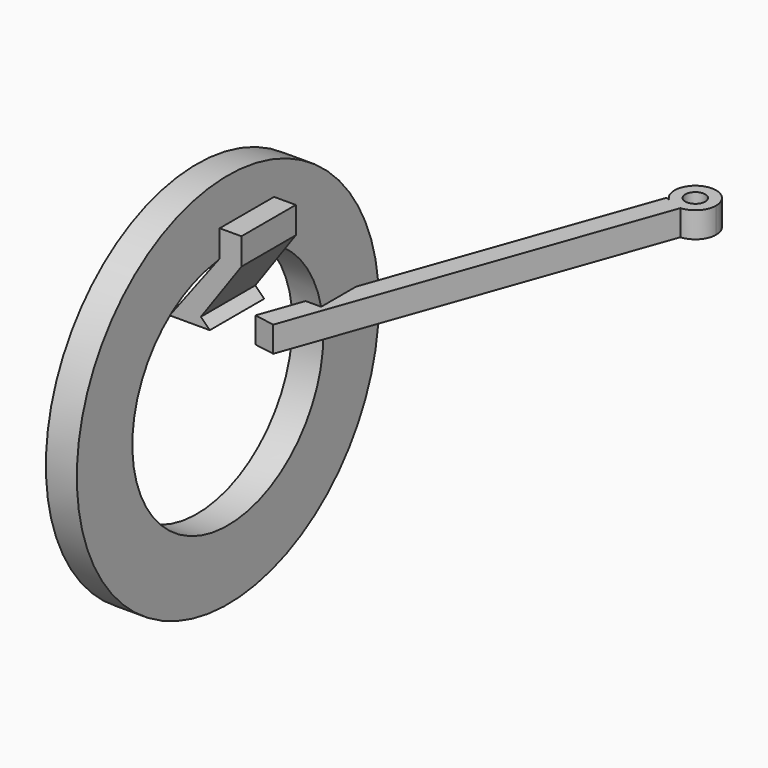
from build123d import *

# Parameters (mm, degrees)
F1_R     = 3.3434072236
F2_DEPTH = 8.636
F0_R     = 63.5
F0_R_2   = 40.1662219946
F3_DEPTH = 10.414
F5_DEPTH = 11.43


# Not quite as in the source:
# - a feature of the source that left no trace in its solid (it failed there, or was rolled back) is left out


with BuildPart() as f2:
    # F1 (on Top) → F2 (new body)
    with BuildSketch(Plane.XY):
        with BuildLine():
            Line((42.4949078619, 144.2979639482), (0, 24.6184635907))
            Line((0, 24.6184635907), (6.9236060732, 23.4437996919))
            Line((6.9236060732, 23.4437996919), (49.013733896, 141.9833076298))
            ThreePointArc((49.013733896, 141.9833076298), (46.1434978735, 142.3662019346), (43.6745030246, 143.8791220613))
            Line((43.6745030246, 143.8791220613), (42.4949078619, 144.2979639482))
        make_face()
        with BuildLine():
            ThreePointArc((55.4755375751, 148.9555081438), (45.7201126941, 155.3787883051), (43.6745030246, 143.8791220613))
            Line((43.6745030246, 143.8791220613), (49.013733896, 141.9833076298))
            ThreePointArc((49.013733896, 141.9833076298), (53.6116733091, 144.2024436904), (55.4755375751, 148.9555081438))
        make_face()
        with Locations((48.4831797689, 148.9555081438)):
            Circle(F1_R, mode=Mode.SUBTRACT)
        with BuildLine():
            Line((49.013733896, 141.9833076298), (43.6745030246, 143.8791220613))
            ThreePointArc((43.6745030246, 143.8791220613), (46.1434978735, 142.3662019346), (49.013733896, 141.9833076298))
        make_face()
    extrude(amount=F2_DEPTH)

    # F0 (on Right) → F3 (join)
    with BuildSketch(Plane.YZ):
        Circle(F0_R)
        Circle(F0_R_2, mode=Mode.SUBTRACT)
    extrude(amount=F3_DEPTH)


with BuildPart() as f5:
    # F4 (on Front) → F5 (new body, symmetric)
    with BuildSketch(Plane.XZ):
        Polygon((13.473616913, 23.2877340168), (10.4794809595, 26.2818709016), (24.1194386035, 45.5774255097), (24.1194386035, 54.5598343015), (16.8004371226, 54.5598343015), (16.8004371226, 45.5774255097), (0, 23.2877340168), align=None)
    extrude(amount=F5_DEPTH, both=True)


solid = Compound([f2.part, f5.part])
